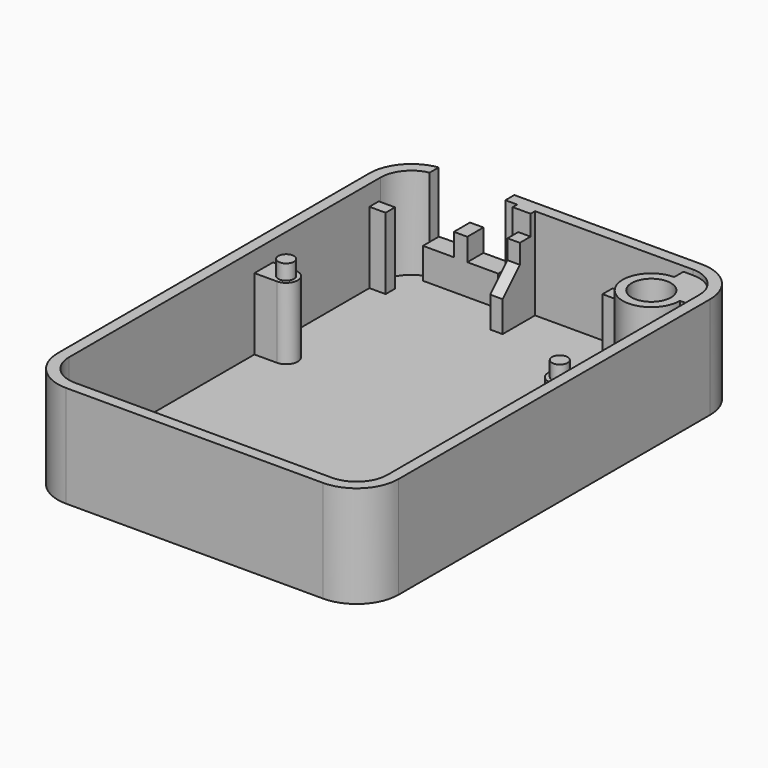
from build123d import *

# Parameters (mm, degrees)
F1_DEPTH    = 18.4
F2_T        = -2
F3_DEPTH    = 0.2
F4_R        = 1.4
F4_W        = 2.9
F4_H        = 2.1
F4_W_2      = 2.2
F4_H_2      = 3.4
F5_DEPTH    = 12.8
F4_R_2      = 3.5
F6_DEPTH    = 15.5
F4_H_3      = 3.85
F7_DEPTH    = 9.5
F8_T4_DEPTH = 22.7734639037
F9_DEPTH    = 1.801
F11_DEPTH   = 1
F10_W       = 1.05
F10_H       = 5.5
F12_DEPTH   = 1.6
F10_H_2     = 10.9
F13_DEPTH   = 3


# Not quite as in the source:
# - a fillet or chamfer that OpenCascade refuses, or shapes differently, is made with other operations: its cross-section is extruded or revolved along the edge and cut away or added


with BuildPart() as f1:
    # F0 (on Top) → F1 (new body)
    with BuildSketch(Plane.XY):
        with BuildLine():
            Line((-22.95, -42.3), (22.95, -42.3))
            ThreePointArc((22.95, -42.3), (28.2533008589, -40.1033008589), (30.45, -34.8))
            Line((30.45, -34.8), (30.45, 34.8))
            ThreePointArc((30.45, 34.8), (28.2533008589, 40.1033008589), (22.95, 42.3))
            Line((22.95, 42.3), (-22.95, 42.3))
            ThreePointArc((-22.95, 42.3), (-28.2533008589, 40.1033008589), (-30.45, 34.8))
            Line((-30.45, 34.8), (-30.45, -34.8))
            ThreePointArc((-30.45, -34.8), (-28.2533008589, -40.1033008589), (-22.95, -42.3))
        make_face()
    extrude(amount=F1_DEPTH)

    # F2
    f2_openings = [f1.faces().sort_by_distance(p)[0] for p in [
        (0, 0, 18.4),
    ]]
    offset(amount=F2_T, openings=f2_openings)

    # F3 (cut): a face of the model
    f3_faces = [f1.faces().sort_by_distance(p)[0] for p in [
        (0, 0, 0),
    ]]
    extrude(f3_faces, amount=-F3_DEPTH, mode=Mode.SUBTRACT)

    # F4 (on face) → F5 (join)
    with BuildSketch(Plane.XY.offset(2)):
        with BuildLine():
            Line((24.45, 6.62), (28.45, 6.62))
            Line((28.45, 6.62), (28.45, 10.78))
            Line((28.45, 10.78), (24.45, 10.78))
            ThreePointArc((24.45, 10.78), (22.37, 8.7), (24.45, 6.62))
        make_face()
        with Locations((24.45, 8.7)):
            Circle(F4_R, mode=Mode.SUBTRACT)
        with BuildLine():
            ThreePointArc((-24.45, 6.62), (-22.37, 8.7), (-24.45, 10.78))
            Line((-24.45, 10.78), (-28.45, 10.78))
            Line((-28.45, 10.78), (-28.45, 6.62))
            Line((-28.45, 6.62), (-24.45, 6.62))
        make_face()
        with Locations((-24.45, 8.7)):
            Circle(F4_R, mode=Mode.SUBTRACT)
        with Locations((-27, 33.35)):
            Rectangle(F4_W, F4_H)
        with Locations((-6.35, 38.6)):
            Rectangle(F4_W_2, F4_H_2)
        with BuildLine():
            ThreePointArc((16.2853761426, 31.995), (16.16, 33.12), (16.2853761426, 34.245))
            Line((16.2853761426, 34.245), (13.45, 34.245))
            Line((13.45, 34.245), (13.45, 31.995))
            Line((13.45, 31.995), (16.2853761426, 31.995))
        make_face()
    extrude(amount=F5_DEPTH)

    # F4 (on face) → F6 (join)
    with BuildSketch(Plane.XY.offset(2)):
        with BuildLine():
            Line((22.95, 40.3), (21.27, 40.3))
            Line((21.27, 40.3), (21.27, 38.23))
            ThreePointArc((21.27, 38.23), (18.0791262952, 37.1112936499), (16.2853761426, 34.245))
            ThreePointArc((16.2853761426, 34.245), (16.16, 33.12), (16.2853761426, 31.995))
            ThreePointArc((16.2853761426, 31.995), (21.835982371, 28.0414407598), (26.38, 33.12))
            Line((26.38, 33.12), (28.45, 33.12))
            Line((28.45, 33.12), (28.45, 34.8))
            ThreePointArc((28.45, 34.8), (26.8390872965, 38.6890872965), (22.95, 40.3))
        make_face()
        with Locations((21.27, 33.12)):
            Circle(F4_R_2, mode=Mode.SUBTRACT)
        with Locations((24.45, 8.7)):
            Circle(F4_R)
        with Locations((-24.45, 8.7)):
            Circle(F4_R)
    extrude(amount=F6_DEPTH)

    # F4 (on face) → F7 (join)
    with BuildSketch(Plane.XY.offset(2)):
        with Locations((-6.35, 34.975)):
            Rectangle(F4_W_2, F4_H_3)
    extrude(amount=F7_DEPTH)

    # F8: chamfer of 4 on 1 edges, made by hand


with BuildPart() as f8_tool2:
    # F8_s3 → F8_t4 (new body)
    with BuildSketch(Plane.YZ.offset(-17.7367319519)):
        Polygon((37.05, 11.5), (33.05, 7.5), (33.05, 11.5), align=None)
    extrude(amount=F8_T4_DEPTH)

    split(bisect_by=Plane.XZ.offset(-36.9), keep=Keep.TOP)


with BuildPart() as f1_1:
    add(f1.part)

    # F8_t1: cut F8_tool2
    add(f8_tool2.part, mode=Mode.SUBTRACT)

    # F4 (on face) → F9 (cut, through all)
    with BuildSketch(Plane.XY.offset(2)):
        with Locations((21.27, 33.12)):
            Circle(F4_R_2)
    extrude(amount=-F9_DEPTH, mode=Mode.SUBTRACT)

    # F10 (on face) → F11 (join)
    with BuildSketch(Plane.XZ.offset(-40.3)):
        Polygon((-8.45, 2), (-7.45, 2), (-7.45, 14.8), (-5.25, 14.8), (-5.25, 18.4), (-8.45, 18.4), align=None)
    extrude(amount=F11_DEPTH)

    # F10 (on face) → F12 (join)
    with BuildSketch(Plane.XZ.offset(-40.3)):
        Polygon((-22.95, 2), (-10.55, 2), (-10.55, 7.5), (-16.075, 7.5), (-16.075, 11.5), (-18.475, 11.5), (-18.475, 7.5), (-22.95, 7.5), align=None)
        with Locations((-23.475, 4.75)):
            Rectangle(F10_W, F10_H)
    extrude(amount=F12_DEPTH)

    # F10 (on face) → F13 (cut, symmetric)
    with BuildSketch(Plane.XZ.offset(-40.3)):
        Polygon((-10.55, 7.5), (-10.55, 18.4), (-22.95, 18.4), (-22.95, 7.5), (-18.475, 7.5), (-18.475, 11.5), (-16.075, 11.5), (-16.075, 7.5), align=None)
        with Locations((-23.475, 12.95)):
            Rectangle(F10_W, F10_H_2)
    extrude(amount=F13_DEPTH, both=True, mode=Mode.SUBTRACT)


solid = f1_1.part
